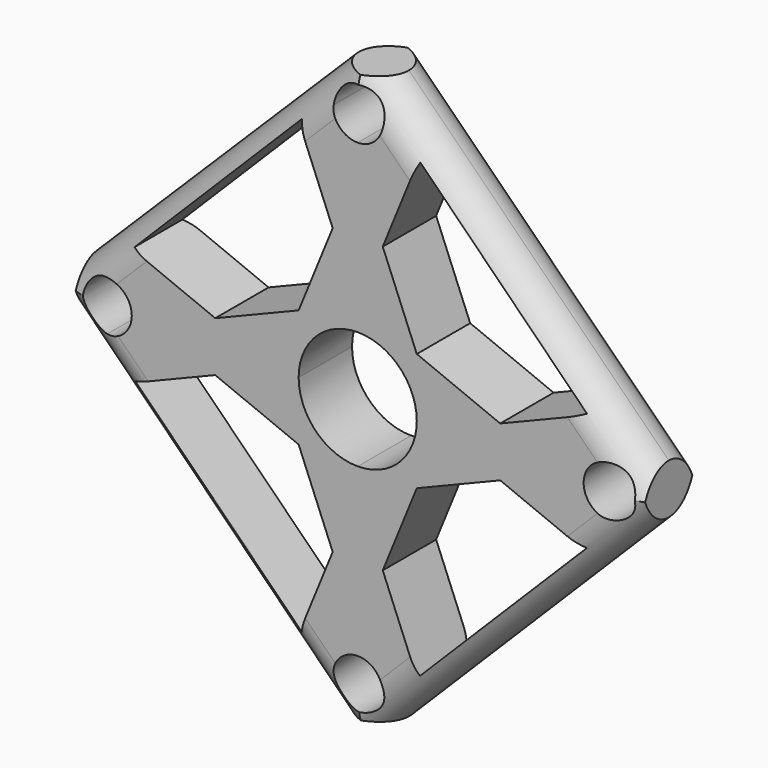
from build123d import *

# Parameters (mm, degrees)
F1_DEPTH    = 20
F2_T1_DEPTH = 159.9071078596
F2_T3_DEPTH = 159.6289321305
F2_T5_DEPTH = 160.2940498067
F2_T7_DEPTH = 159.881620562
F3_T1_DEPTH = 160.2940498067
F3_T3_DEPTH = 159.881620562
F3_T5_DEPTH = 159.6289321305
F3_T7_DEPTH = 159.9071078596


# Not quite as in the source:
# - a fillet or chamfer that OpenCascade refuses, or shapes differently, is made with other operations: its cross-section is extruded or revolved along the edge and cut away or added


with BuildPart() as f1:
    # F0 (on Front) → F1 (new body)
    with BuildSketch(Plane.XZ):
        with BuildLine():
            ThreePointArc((-17.6980390272, 0), (-12.5144034098, 12.5144034098), (0, 17.6980390272))
            Line((0, 17.6980390272), (0, 67.6980390272))
            ThreePointArc((0, 67.6980390272), (-5.263032473, 69.8547732479), (-7.4991416822, 75.0845752437))
            Line((-7.4991416822, 75.0845752437), (-7.6504267269, 85.08343082))
            Line((-7.6504267269, 85.08343082), (-17.6980390272, 67.6980390272))
            Line((-17.6980390272, 67.6980390272), (-7.5, 42.6980390272))
            Line((-7.5, 42.6980390272), (-17.6980390272, 17.6980390272))
            Line((-17.6980390272, 17.6980390272), (-42.6980390272, 7.5))
            Line((-42.6980390272, 7.5), (-67.6980390272, 17.6980390272))
            Line((-67.6980390272, 17.6980390272), (-85.443013147, 7.8382610153))
            Line((-85.443013147, 7.8382610153), (-85.443013147, -7.1617389847))
            Line((-85.443013147, -7.1617389847), (-75.4485949977, -7.495813612))
            ThreePointArc((-75.4485949977, -7.495813612), (-80.4120025014, 5.3911580286), (-67.6980390272, 0))
            Line((-67.6980390272, 0), (-17.6980390272, 0))
        make_face()
        with BuildLine():
            Line((0, -31.6828936338), (0, -17.6980390272))
            ThreePointArc((0, -17.6980390272), (-12.5144034098, -12.5144034098), (-17.6980390272, 0))
            Line((-17.6980390272, 0), (-67.6980390272, 0))
            ThreePointArc((-67.6980390272, 0), (-69.984075553, -5.3911580286), (-75.4485949977, -7.495813612))
            Line((-75.4485949977, -7.495813612), (-85.443013147, -7.1617389847))
            Line((-85.443013147, -7.1617389847), (-67.6980390272, -17.6980390272))
            Line((-67.6980390272, -17.6980390272), (-42.6980390272, -7.5))
            Line((-42.6980390272, -7.5), (-17.6980390272, -17.6980390272))
            Line((-17.6980390272, -17.6980390272), (-7.5, -42.6980390272))
            Line((-7.5, -42.6980390272), (-17.6980390272, -67.6980390272))
            Line((-17.6980390272, -67.6980390272), (-7.5, -85.1980390272))
            Line((-7.5, -85.1980390272), (-7.5, -75.1980390272))
            ThreePointArc((-7.5, -75.1980390272), (-5.3033008589, -69.8947381683), (0, -67.6980390272))
            Line((0, -67.6980390272), (0, -31.6828936338))
        make_face()
        with BuildLine():
            Line((67.6980390272, 0), (17.6980390272, 0))
            ThreePointArc((17.6980390272, 0), (12.5144034098, -12.5144034098), (0, -17.6980390272))
            Line((0, -17.6980390272), (0, -31.6828936338))
            Line((0, -31.6828936338), (0, -67.6980390272))
            ThreePointArc((0, -67.6980390272), (5.3033008589, -69.8947381683), (7.5, -75.1980390272))
            ThreePointArc((7.5, -75.1980390272), (0, -82.6980390272), (-7.5, -75.1980390272))
            Line((-7.5, -75.1980390272), (-7.5, -85.1980390272))
            Line((-7.5, -85.1980390272), (7.5, -85.1980390272))
            Line((7.5, -85.1980390272), (17.6980390272, -67.6980390272))
            Line((17.6980390272, -67.6980390272), (7.5, -42.6980390272))
            Line((7.5, -42.6980390272), (17.6980390272, -17.6980390272))
            Line((17.6980390272, -17.6980390272), (42.6980390272, -7.5))
            Line((42.6980390272, -7.5), (67.6980390272, -17.6980390272))
            Line((67.6980390272, -17.6980390272), (85.1980390272, -7.5))
            Line((85.1980390272, -7.5), (75.1980390272, -7.5))
            ThreePointArc((75.1980390272, -7.5), (69.8947381683, -5.3033008589), (67.6980390272, 0))
        make_face()
        with BuildLine():
            ThreePointArc((0, 17.6980390272), (12.5144034098, 12.5144034098), (17.6980390272, 0))
            Line((17.6980390272, 0), (67.6980390272, 0))
            ThreePointArc((67.6980390272, 0), (75.1980390272, 7.5), (82.6980390272, 0))
            ThreePointArc((82.6980390272, 0), (80.5013398861, -5.3033008589), (75.1980390272, -7.5))
            Line((75.1980390272, -7.5), (85.1980390272, -7.5))
            Line((85.1980390272, -7.5), (85.1980390272, 7.5))
            Line((85.1980390272, 7.5), (67.6980390272, 17.6980390272))
            Line((67.6980390272, 17.6980390272), (42.6980390272, 7.5))
            Line((42.6980390272, 7.5), (17.6980390272, 17.6980390272))
            Line((17.6980390272, 17.6980390272), (7.5, 42.6980390272))
            Line((7.5, 42.6980390272), (17.6980390272, 67.6980390272))
            Line((17.6980390272, 67.6980390272), (7.3495732731, 85.08343082))
            Line((7.3495732731, 85.08343082), (-7.6504267269, 85.08343082))
            Line((-7.6504267269, 85.08343082), (-7.4991416822, 75.0845752437))
            ThreePointArc((-7.4991416822, 75.0845752437), (-0.0567335149, 82.6978244447), (7.5, 75.1980390272))
            ThreePointArc((7.5, 75.1980390272), (5.3033008589, 69.8947381683), (0, 67.6980390272))
            Line((0, 67.6980390272), (0, 17.6980390272))
        make_face()
        Polygon((67.6980390272, 17.6980390272), (85.1980390272, 7.5), (7.3495732731, 85.08343082), (17.6980390272, 67.6980390272), align=None)
        Polygon((-17.6980390272, 67.6980390272), (-7.6504267269, 85.08343082), (-85.443013147, 7.8382610153), (-67.6980390272, 17.6980390272), align=None)
        Polygon((-67.6980390272, -17.6980390272), (-85.443013147, -7.1617389847), (-7.5, -85.1980390272), (-17.6980390272, -67.6980390272), align=None)
        Polygon((7.5, -85.1980390272), (85.1980390272, -7.5), (67.6980390272, -17.6980390272), (17.6980390272, -67.6980390272), align=None)
    extrude(amount=F1_DEPTH)

    # F2: fillet of radius 10 on 4 edges, made by hand

    # F2_s2 → F2_t1 (cut)
    with BuildSketch(Plane(origin=(56.7021033547, 0, -56.5090611659), x_dir=(0, 1, 0), z_dir=(-0.7083114757, 0, 0.7059000308))):
        with BuildLine():
            ThreePointArc((-10, -65.4536344384), (-17.0710678119, -62.5247022502), (-20, -55.4536344384))
            Line((-20, -55.4536344384), (-20, -65.4536344384))
            Line((-20, -65.4536344384), (-10, -65.4536344384))
        make_face()
    extrude(amount=F2_T1_DEPTH, mode=Mode.SUBTRACT)

    # F2_s4 → F2_t3 (cut)
    with BuildSketch(Plane(origin=(56.4284054026, 0, 56.0313258334), x_dir=(0, 1, 0), z_dir=(-0.709599053, 0, -0.704605694))):
        with BuildLine():
            ThreePointArc((-10, -65.7656561682), (-17.0710678119, -62.83672398), (-20, -55.7656561682))
            Line((-20, -55.7656561682), (-20, -65.7656561682))
            Line((-20, -65.7656561682), (-10, -65.7656561682))
        make_face()
    extrude(amount=F2_T3_DEPTH, mode=Mode.SUBTRACT)

    # F2_s6 → F2_t5 (cut)
    with BuildSketch(Plane(origin=(-56.7566324146, 0, 56.8245621728), x_dir=(0, 1, 0), z_dir=(0.7066837539, 0, -0.7075295556))):
        with BuildLine():
            ThreePointArc((-10, -65.514541709), (-17.0710678119, -62.5856095209), (-20, -55.514541709))
            Line((-20, -55.514541709), (-20, -65.514541709))
            Line((-20, -65.514541709), (-10, -65.514541709))
        make_face()
    extrude(amount=F2_T5_DEPTH, mode=Mode.SUBTRACT)

    # F2_s8 → F2_t7 (cut)
    with BuildSketch(Plane(origin=(-56.5266890433, 0, -56.5266890433), x_dir=(0, 1, 0), z_dir=(0.7071067812, 0, 0.7071067812))):
        with BuildLine():
            ThreePointArc((-10, -65.5474119988), (-17.0710678119, -62.6184798107), (-20, -55.5474119988))
            Line((-20, -55.5474119988), (-20, -65.5474119988))
            Line((-20, -65.5474119988), (-10, -65.5474119988))
        make_face()
    extrude(amount=F2_T7_DEPTH, mode=Mode.SUBTRACT)

    # F3: fillet of radius 10 on 4 edges, made by hand

    # F3_s2 → F3_t1 (cut)
    with BuildSketch(Plane(origin=(-56.7566324146, 0, 56.8245621728), x_dir=(0, 1, 0), z_dir=(0.7066837539, 0, -0.7075295556))):
        with BuildLine():
            ThreePointArc((0, -55.514541709), (-2.9289321881, -62.5856095209), (-10, -65.514541709))
            Line((-10, -65.514541709), (0, -65.514541709))
            Line((0, -65.514541709), (0, -55.514541709))
        make_face()
    extrude(amount=F3_T1_DEPTH, mode=Mode.SUBTRACT)

    # F3_s4 → F3_t3 (cut)
    with BuildSketch(Plane(origin=(-56.5266890433, 0, -56.5266890433), x_dir=(0, 1, 0), z_dir=(0.7071067812, 0, 0.7071067812))):
        with BuildLine():
            ThreePointArc((0, -55.5474119988), (-2.9289321881, -62.6184798107), (-10, -65.5474119988))
            Line((-10, -65.5474119988), (0, -65.5474119988))
            Line((0, -65.5474119988), (0, -55.5474119988))
        make_face()
    extrude(amount=F3_T3_DEPTH, mode=Mode.SUBTRACT)

    # F3_s6 → F3_t5 (cut)
    with BuildSketch(Plane(origin=(56.4284054026, 0, 56.0313258334), x_dir=(0, 1, 0), z_dir=(-0.709599053, 0, -0.704605694))):
        with BuildLine():
            ThreePointArc((0, -55.7656561682), (-2.9289321881, -62.83672398), (-10, -65.7656561682))
            Line((-10, -65.7656561682), (0, -65.7656561682))
            Line((0, -65.7656561682), (0, -55.7656561682))
        make_face()
    extrude(amount=F3_T5_DEPTH, mode=Mode.SUBTRACT)

    # F3_s8 → F3_t7 (cut)
    with BuildSketch(Plane(origin=(56.7021033547, 0, -56.5090611659), x_dir=(0, 1, 0), z_dir=(-0.7083114757, 0, 0.7059000308))):
        with BuildLine():
            ThreePointArc((0, -55.4536344384), (-2.9289321881, -62.5247022502), (-10, -65.4536344384))
            Line((-10, -65.4536344384), (0, -65.4536344384))
            Line((0, -65.4536344384), (0, -55.4536344384))
        make_face()
    extrude(amount=F3_T7_DEPTH, mode=Mode.SUBTRACT)


solid = f1.part
